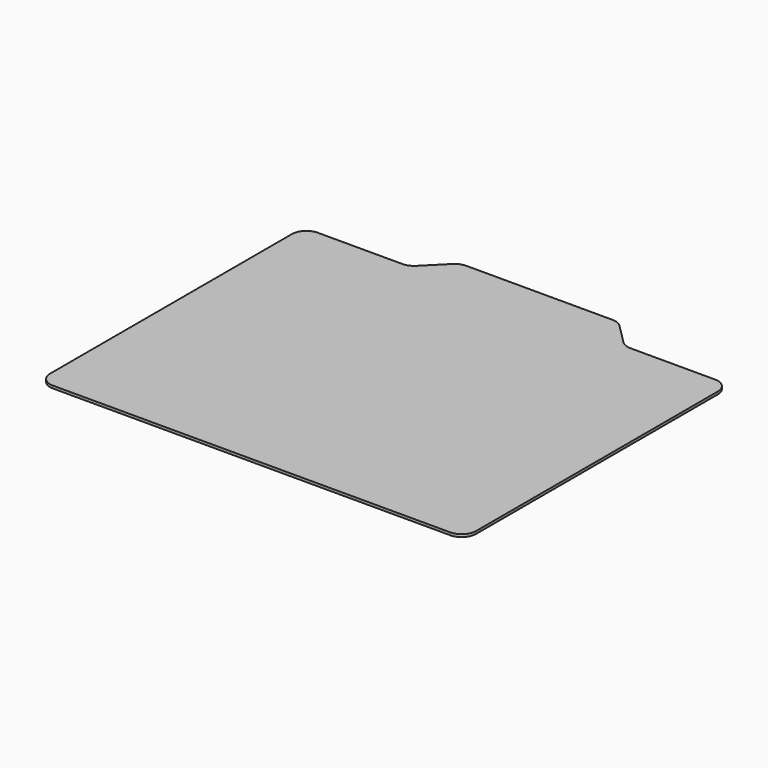
from build123d import *

# Parameters (mm, degrees)
F1_DEPTH = 0.9
F2_R     = 5


# Not quite as in the source:
# - a feature names something its author has since deleted; it is built from what else it names


with BuildPart() as f1:
    # F0 (on Top) → F1 (new body)
    with BuildSketch(Plane.XY):
        Polygon((-74, -59.5467374876), (74, -59.5467374876), (74, 55.4532625124), (37.5, 55.4532625124), (27.5, 65.4532625124), (-27.5, 65.4532625124), (-37.5, 55.4532625124), (-74, 55.4532625124), align=None)
    extrude(amount=F1_DEPTH)

    # F2
    f2_edges = [f1.edges().sort_by_distance(p)[0] for p in [
        (37.5, 55.453263, 0.45),
        (27.5, 65.453263, 0.45),
        (-37.5, 55.453263, 0.45),
        (-27.5, 65.453263, 0.45),
        (-74, 55.453263, 0.45),
        (-74, -59.546737, 0.45),
        (74, -59.546737, 0.45),
        (74, 55.453263, 0.45),
    ]]
    fillet(f2_edges, radius=F2_R)


solid = f1.part
